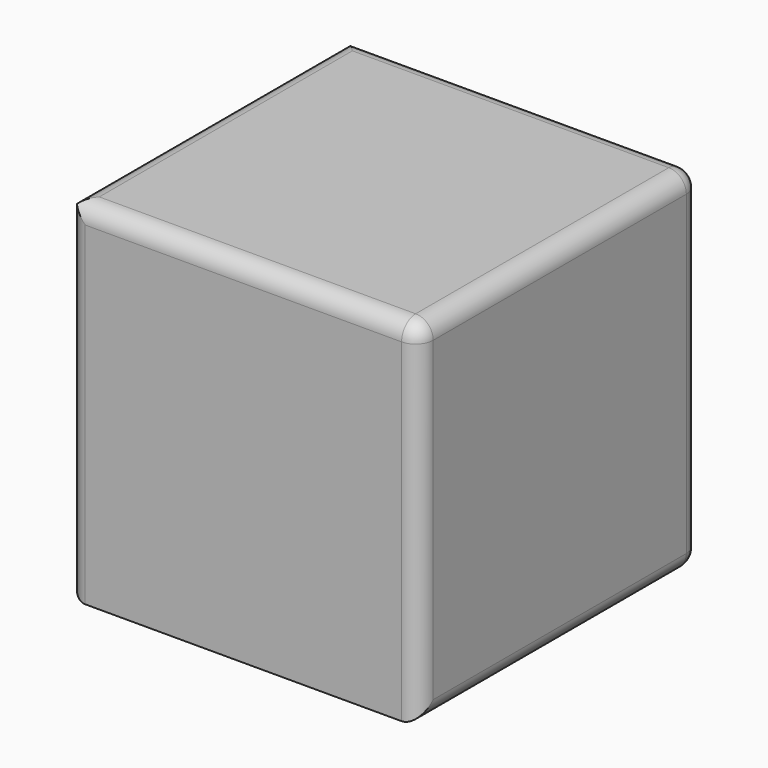
from build123d import *

# Parameters (mm, degrees)
F0_W         = 50.8
F0_H         = 50.8
F1_DEPTH     = 50.8
F2_R         = 2.54
F3_T1_DEPTH  = 52.07
F3_T3_DEPTH  = 45.72
F3_T5_DEPTH  = 54.61
F3_T7_DEPTH  = 45.72
F3_T9_DEPTH  = 54.61
F3_S13_W     = 2.5908
F3_S13_H     = 2.5908
F3_T14_DEPTH = 2.5908
F3_S19_W     = 2.5908
F3_S19_H     = 2.5908
F3_T20_DEPTH = 2.5908
F3_S25_W     = 2.5908
F3_S25_H     = 2.5908
F3_T26_DEPTH = 2.5908


# Not quite as in the source:
# - a fillet or chamfer that OpenCascade refuses, or shapes differently, is made with other operations: its cross-section is extruded or revolved along the edge and cut away or added


with BuildPart() as f1:
    # F0 (on Top) → F1 (new body)
    with BuildSketch(Plane.XY):
        Rectangle(F0_W, F0_H)
    extrude(amount=F1_DEPTH)

    # F2
    f2_edges = [f1.edges().sort_by_distance(p)[0] for p in [
        (-25.4, 25.4, 25.4),
        (-25.4, -25.4, 25.4),
        (-25.4, 0, 0),
        (-25.4, 0, 50.8),
    ]]
    fillet(f2_edges, radius=F2_R)

    # F3: fillet of radius 2.54 on 9 edges, made by hand

    # F3_s2 → F3_t1 (cut)
    with BuildSketch(Plane.YZ.offset(-29.21)):
        with BuildLine():
            ThreePointArc((25.4, 48.26), (24.6560512242, 50.0560512242), (22.86, 50.8))
            Line((22.86, 50.8), (25.4, 50.8))
            Line((25.4, 50.8), (25.4, 48.26))
        make_face()
        with BuildLine():
            ThreePointArc((-22.86, 50.8), (-24.6560512242, 50.0560512242), (-25.4, 48.26))
            Line((-25.4, 48.26), (-25.4, 50.8))
            Line((-25.4, 50.8), (-22.86, 50.8))
        make_face()
        with BuildLine():
            ThreePointArc((25.4, 2.54), (24.6560512242, 0.7439487758), (22.86, 0))
            Line((22.86, 0), (25.4, 0))
            Line((25.4, 0), (25.4, 2.54))
        make_face()
    extrude(amount=F3_T1_DEPTH, mode=Mode.SUBTRACT)

    # F3_s4 → F3_t3 (cut)
    with BuildSketch(Plane.XZ.offset(-22.86)):
        with BuildLine():
            ThreePointArc((25.4, 48.26), (24.6560512242, 50.0560512242), (22.86, 50.8))
            Line((22.86, 50.8), (25.4, 50.8))
            Line((25.4, 50.8), (25.4, 48.26))
        make_face()
    extrude(amount=F3_T3_DEPTH, mode=Mode.SUBTRACT)

    # F3_s6 → F3_t5 (cut)
    with BuildSketch(Plane.XY.offset(-6.35)):
        with BuildLine():
            ThreePointArc((25.4, -22.86), (24.6560512242, -24.6560512242), (22.86, -25.4))
            Line((22.86, -25.4), (25.4, -25.4))
            Line((25.4, -25.4), (25.4, -22.86))
        make_face()
    extrude(amount=F3_T5_DEPTH, mode=Mode.SUBTRACT)

    # F3_s8 → F3_t7 (cut)
    with BuildSketch(Plane.XY.offset(2.54)):
        with BuildLine():
            ThreePointArc((22.86, 25.4), (24.6560512242, 24.6560512242), (25.4, 22.86))
            Line((25.4, 22.86), (25.4, 25.4))
            Line((25.4, 25.4), (22.86, 25.4))
        make_face()
    extrude(amount=F3_T7_DEPTH, mode=Mode.SUBTRACT)

    # F3_s10 → F3_t9 (cut)
    with BuildSketch(Plane.XZ.offset(-22.86)):
        with BuildLine():
            ThreePointArc((22.86, 0), (24.6560512242, 0.7439487758), (25.4, 2.54))
            Line((25.4, 2.54), (25.4, 0))
            Line((25.4, 0), (22.86, 0))
        make_face()
    extrude(amount=F3_T9_DEPTH, mode=Mode.SUBTRACT)


with BuildPart() as f3_tool12:
    # F3_s13 → F3_t14 (new body)
    with BuildSketch(Plane.XZ.offset(-22.86)):
        with Locations((24.1554, 49.5554)):
            Rectangle(F3_S13_W, F3_S13_H)
    extrude(amount=-F3_T14_DEPTH)

    # F3_s15 → F3_t16 (revolve, cut)
    with BuildSketch(Plane(origin=(22.86, 22.86, 48.26), x_dir=(-0.7071067812, 0, -0.7071067812), z_dir=(0.7071067812, 0, -0.7071067812))):
        with BuildLine():
            ThreePointArc((0, -2.54), (2.54, 0), (0, 2.54))
            Line((0, 2.54), (0, -2.54))
        make_face()
    revolve(axis=Axis((22.86, 22.86, 48.26), (0, 1, 0)), mode=Mode.SUBTRACT)


with BuildPart() as f1_1:
    add(f1.part)

    # F3_t11: cut F3_tool12
    add(f3_tool12.part, mode=Mode.SUBTRACT)


with BuildPart() as f3_tool18:
    # F3_s19 → F3_t20 (new body)
    with BuildSketch(Plane.YZ.offset(22.86)):
        with Locations((-24.1554, 49.5554)):
            Rectangle(F3_S19_W, F3_S19_H)
    extrude(amount=F3_T20_DEPTH)

    # F3_s21 → F3_t22 (revolve, cut)
    with BuildSketch(Plane(origin=(22.86, -22.86, 48.26), x_dir=(0, 0.7071067812, -0.7071067812), z_dir=(0, -0.7071067812, -0.7071067812))):
        with BuildLine():
            ThreePointArc((0, -2.54), (2.54, 0), (0, 2.54))
            Line((0, 2.54), (0, -2.54))
        make_face()
    revolve(axis=Axis((22.86, -22.86, 48.26), (1, 0, 0)), mode=Mode.SUBTRACT)


with BuildPart() as f1_2:
    add(f1_1.part)

    # F3_t17: cut F3_tool18
    add(f3_tool18.part, mode=Mode.SUBTRACT)


with BuildPart() as f3_tool24:
    # F3_s25 → F3_t26 (new body)
    with BuildSketch(Plane.XZ.offset(-22.86)):
        with Locations((24.1554, 1.2446)):
            Rectangle(F3_S25_W, F3_S25_H)
    extrude(amount=-F3_T26_DEPTH)

    # F3_s27 → F3_t28 (revolve, cut)
    with BuildSketch(Plane(origin=(22.86, 22.86, 2.54), x_dir=(-0.7071067812, 0, 0.7071067812), z_dir=(-0.7071067812, 0, -0.7071067812))):
        with BuildLine():
            ThreePointArc((0, -2.54), (2.54, 0), (0, 2.54))
            Line((0, 2.54), (0, -2.54))
        make_face()
    revolve(axis=Axis((22.86, 22.86, 2.54), (0, 1, 0)), mode=Mode.SUBTRACT)


with BuildPart() as f1_3:
    add(f1_2.part)

    # F3_t23: cut F3_tool24
    add(f3_tool24.part, mode=Mode.SUBTRACT)


solid = f1_3.part
